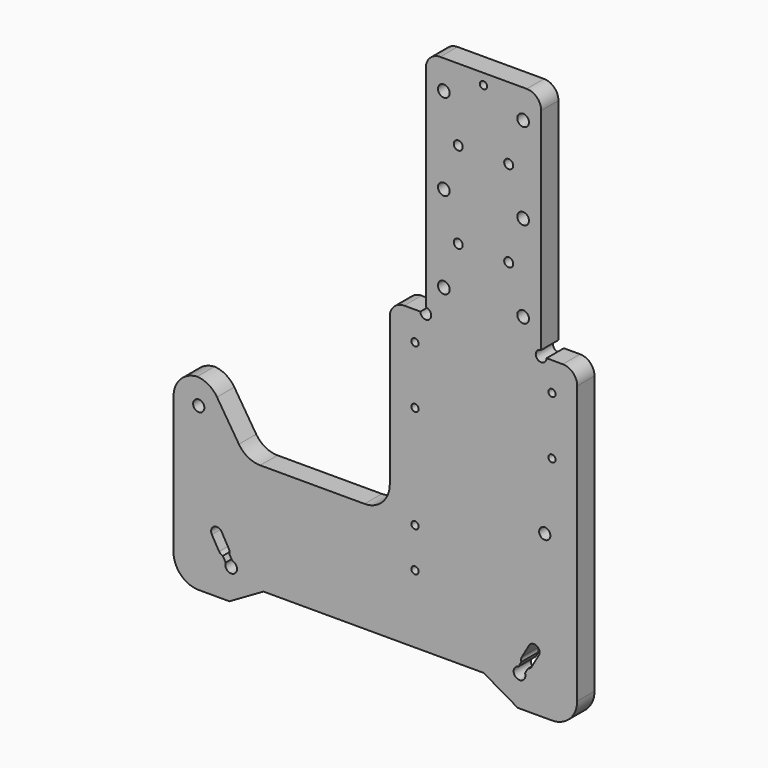
from build123d import *

# Parameters (mm, degrees)
F0_R     = 4.953
F0_R_2   = 3.175
F0_R_3   = 5.1562
F0_R_4   = 3.96875
F1_DEPTH = 19.05


# Not quite as in the source:
# - ends of sketch curves that miss each other by under 0.0002 mm in the source are joined


with BuildPart() as f1:
    # F0 (on Front) → F1 (new body)
    with BuildSketch(Plane.XZ):
        with BuildLine():
            ThreePointArc((177.8, 25.4), (174.0802561211, 34.3802561211), (165.1, 38.1))
            Line((165.1, 38.1), (150.8125, 38.1))
            ThreePointArc((150.8125, 38.1), (142.6824039546, 34.7324039546), (146.05, 42.8625))
            Line((146.05, 42.8625), (146.05, 228.6))
            ThreePointArc((146.05, 228.6), (142.3302561211, 237.5802561211), (133.35, 241.3))
            Line((133.35, 241.3), (57.15, 241.3))
            ThreePointArc((57.15, 241.3), (48.1697438789, 237.5802561211), (44.45, 228.6))
            Line((44.45, 228.6), (44.45, 42.8625))
            ThreePointArc((44.45, 42.8625), (47.8175960454, 34.7324039546), (39.6875, 38.1))
            Line((39.6875, 38.1), (25.4, 38.1))
            ThreePointArc((25.4, 38.1), (16.4197438789, 34.3802561211), (12.7, 25.4))
            Line((12.7, 25.4), (12.7, -104.775))
            ThreePointArc((12.7, -104.775), (6.1904482119, -120.4904482119), (-9.525, -127))
            Line((-9.525, -127), (-101.4522228, -127))
            ThreePointArc((-101.4522228, -127), (-112.1350976667, -124.2641459429), (-120.1878905046, -116.7301403448))
            Line((-120.1878905046, -116.7301403448), (-139.4968508, -86.469855))
            ThreePointArc((-139.4968508, -86.469855), (-146.9715660509, -79.2640655101), (-156.9037505938, -76.2397575751))
            ThreePointArc((-156.9037505938, -76.2397575751), (-171.7534129546, -83.1865755647), (-177.8, -98.425))
            Line((-177.8, -98.425), (-177.8, -219.075))
            ThreePointArc((-177.8, -219.075), (-171.2904482119, -234.7904482119), (-155.575, -241.3))
            Line((-155.575, -241.3), (-128.5875, -241.3))
            Line((-128.5875, -241.3), (-98.5712024, -223.970088))
            Line((-98.5712024, -223.970088), (95.3962024, -223.970088))
            Line((95.3962024, -223.970088), (125.4125, -241.3))
            Line((125.4125, -241.3), (155.575, -241.3))
            ThreePointArc((155.575, -241.3), (171.2904482119, -234.7904482119), (177.8, -219.075))
            Line((177.8, -219.075), (177.8, 25.4))
        make_face()
        with BuildLine():
            Line((-137.639425, -205.5625302), (-143.989425, -194.564))
            ThreePointArc((-143.989425, -194.564), (-142.1764994912, -187.7980758813), (-135.4105758813, -189.6110005088))
            Line((-135.4105758813, -189.6110005088), (-129.060575, -200.6095302))
            ThreePointArc((-129.060575, -200.6095302), (-128.4232829137, -202.5764541494), (-128.6445091035, -204.6321752201))
            Line((-128.6445091035, -204.6321752201), (-126.1204742, -209.0039))
            ThreePointArc((-126.1204742, -209.0039), (-124.4219046114, -218.5499378494), (-131.8397164566, -212.3058998322))
            Line((-131.8397164566, -212.3058998322), (-134.3637394, -207.934179))
            ThreePointArc((-134.3637394, -207.934179), (-136.2546626338, -207.0979055699), (-137.639425, -205.5625302))
        make_face(mode=Mode.SUBTRACT)
        with Locations((-155.575, -98.425)):
            Circle(F0_R, mode=Mode.SUBTRACT)
        with Locations((34.925, -164.051488)):
            Circle(F0_R_2, mode=Mode.SUBTRACT)
        with Locations((34.925, -129.126488)):
            Circle(F0_R_2, mode=Mode.SUBTRACT)
        with BuildLine():
            Line((129.060575, -200.6095302), (135.410575, -189.611))
            ThreePointArc((135.410575, -189.611), (142.1764994912, -187.7980758813), (143.9894241187, -194.5639994912))
            Line((143.9894241187, -194.5639994912), (137.639425, -205.5625302))
            ThreePointArc((137.639425, -205.5625302), (136.2546626338, -207.0979055699), (134.3637392893, -207.9341784706))
            Line((134.3637392893, -207.9341784706), (131.839716, -212.3059))
            ThreePointArc((131.839716, -212.3059), (124.4219046114, -218.5499378494), (126.1204745175, -209.0039018342))
            Line((126.1204745175, -209.0039018342), (128.6444976, -204.632179))
            ThreePointArc((128.6444976, -204.632179), (128.4232829137, -202.5764541494), (129.060575, -200.6095302))
        make_face(mode=Mode.SUBTRACT)
        with Locations((34.925, -38.1)):
            Circle(F0_R_2, mode=Mode.SUBTRACT)
        with Locations((149.225, -98.425)):
            Circle(F0_R, mode=Mode.SUBTRACT)
        with Locations((155.575, -38.1)):
            Circle(F0_R_2, mode=Mode.SUBTRACT)
        with Locations((34.925, 12.7)):
            Circle(F0_R_2, mode=Mode.SUBTRACT)
        with Locations((60.325, 63.5)):
            Circle(F0_R_3, mode=Mode.SUBTRACT)
        with Locations((73.025, 101.6)):
            Circle(F0_R_4, mode=Mode.SUBTRACT)
        with Locations((155.575, 12.7)):
            Circle(F0_R_2, mode=Mode.SUBTRACT)
        with Locations((130.175, 63.5)):
            Circle(F0_R_3, mode=Mode.SUBTRACT)
        with Locations((117.475, 101.6)):
            Circle(F0_R_4, mode=Mode.SUBTRACT)
        with Locations((60.325, 139.7)):
            Circle(F0_R_3, mode=Mode.SUBTRACT)
        with Locations((73.025, 177.8)):
            Circle(F0_R_4, mode=Mode.SUBTRACT)
        with Locations((60.325, 215.9)):
            Circle(F0_R_3, mode=Mode.SUBTRACT)
        with Locations((130.175, 139.7)):
            Circle(F0_R_3, mode=Mode.SUBTRACT)
        with Locations((117.475, 177.8)):
            Circle(F0_R_4, mode=Mode.SUBTRACT)
        with Locations((95.25, 231.775)):
            Circle(F0_R_2, mode=Mode.SUBTRACT)
        with Locations((130.175, 215.9)):
            Circle(F0_R_3, mode=Mode.SUBTRACT)
    extrude(amount=F1_DEPTH)


solid = f1.part
